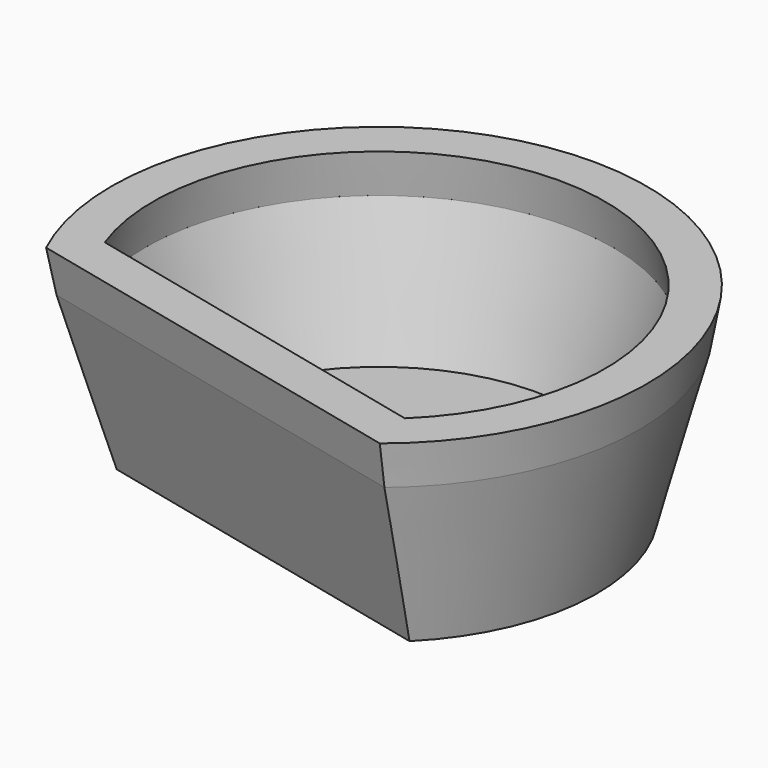
from build123d import *

# Parameters (mm, degrees)
F1_DEPTH               = 46.99
DRAFT_F1_DRAFTED_ANGLE = -15
F2_T                   = 7.62
F3_DEPTH               = 12.7
DRAFT_F3_DRAFTED_ANGLE = -10


# Not quite as in the source:
# - an extrude with a draft is written as a straight extrude whose walls are then drafted
# - a shell that OpenCascade refuses in one call is made with other operations: the cavity is built on its own and cut out


with BuildPart() as f1:
    # F0 (on Top) → F1 (new body)
    with BuildSketch(Plane.XY):
        with BuildLine():
            Line((-183.3270404259, 24.9811097347), (-76.2827530062, 0))
            ThreePointArc((-76.2827530062, 0), (-107.2916058627, 108.9602154415), (-183.3270404259, 24.9811097347))
        make_face()
    extrude(amount=F1_DEPTH)

    # draft_F1_drafted
    draft_f1_drafted_walls = [f1.faces().sort_by_distance(p)[0] for p in [
        (-129.8048967161, 12.4905548673, 31.3266666667),
        (-107.2916058627, 108.9602154415, 31.3266666667),
    ]]
    draft(draft_f1_drafted_walls, neutral_plane=Plane.XY, angle=DRAFT_F1_DRAFTED_ANGLE)

    # F2: shell of thickness 7.62, made by hand


with BuildPart() as f2_core1:
    # F2_t2: copy of F1
    add(f1.part)

    # the walls: a layer under each face that stays
    f2_faces = [f2_core1.faces().sort_by_distance(p)[0] for p in [
        (-131.2356362985, 6.3598224574, 23.495),
        (-105.8608662803, 115.0909478514, 23.495),
        (-122.013181448, 55.3276211654, 0),
    ]]
    thicken(f2_faces, amount=-F2_T, mode=Mode.SUBTRACT)


with BuildPart() as f1_1:
    add(f1.part)

    # what is left inside the walls is the cavity
    f2_cavity = [f2_core1.part.solids().sort_by_distance(p)[0] for p in [
        (-122.013181, 35.013436, 46.9138),
    ]]
    add(f2_cavity, mode=Mode.SUBTRACT)


with BuildPart() as f3_drafted:
    # F3 (new): a face of the model
    f3_faces = [f1_1.part.faces().sort_by_distance(p)[0] for p in [
        (-132.1966802726, 2.2417400951, 46.99),
    ]]
    extrude(f3_faces, amount=F3_DEPTH)

    # draft_F3_drafted
    draft_f3_drafted_walls = [f3_drafted.faces().sort_by_distance(p)[0] for p in [
        (-132.6663758809, 0.2290900476, 55.4566666667),
        (-104.4301266978, 121.2216802613, 55.4566666667),
        (-130.8735261771, 7.9114676935, 55.4566666667),
        (-106.2229764017, 113.5393026153, 55.4566666667),
    ]]
    draft(draft_f3_drafted_walls, neutral_plane=Plane(origin=(-120.1436487753, 53.8890920975, 46.99), x_dir=(1, 0, 0), z_dir=(0, 0, 1)), angle=DRAFT_F3_DRAFTED_ANGLE)


with BuildPart() as f1_2:
    add(f1_1.part)

    # join_F3_drafted: union F3_drafted
    add(f3_drafted.part)


solid = f1_2.part
